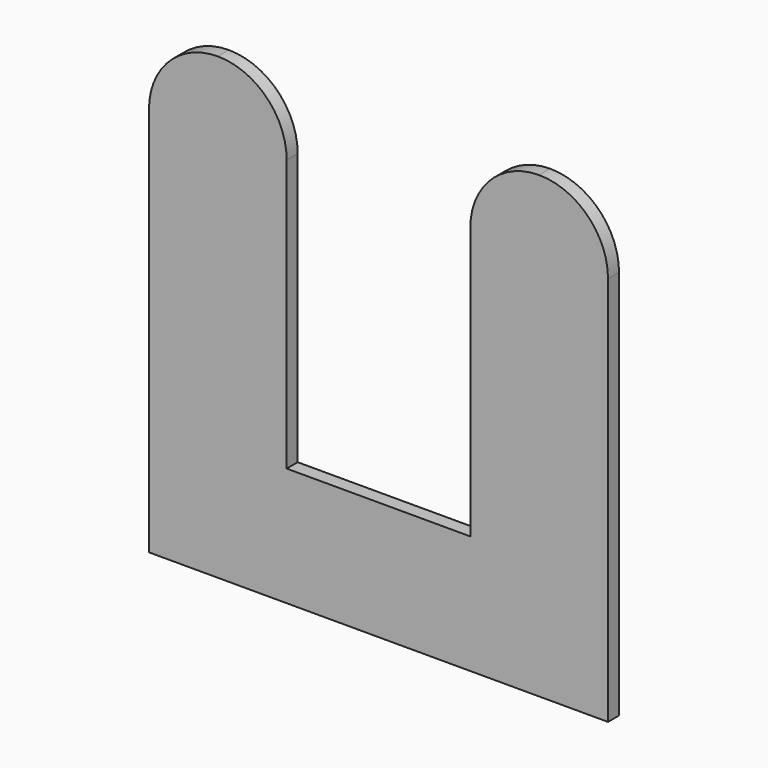
from build123d import *

# Parameters (mm, degrees)
F1_DEPTH = 3
F2_R     = 14.99999


# Not quite as in the source:
# - a fillet or chamfer is up to 0.001 mm smaller than in the source, because OpenCascade refuses the exact size


with BuildPart() as f1:
    # F0 (on Front) → F1 (new body)
    with BuildSketch(Plane.XZ):
        Polygon((0, 25.8250685402), (0, 0), (100, 0), (100, 25.8250685402), (100, 100), (70, 100), (70, 25.8250685402), (30, 25.8250685402), (30, 100), (0, 100), align=None)
    extrude(amount=F1_DEPTH)

    # F2 (radius 15 in the source; OpenCascade refuses exactly that, so slightly less here)
    f2_edges = [f1.edges().sort_by_distance(p)[0] for p in [
        (100, -1.5, 100),
        (70, -1.5, 100),
        (30, -1.5, 100),
        (0, -1.5, 100),
    ]]
    fillet(f2_edges, radius=F2_R)


solid = f1.part
